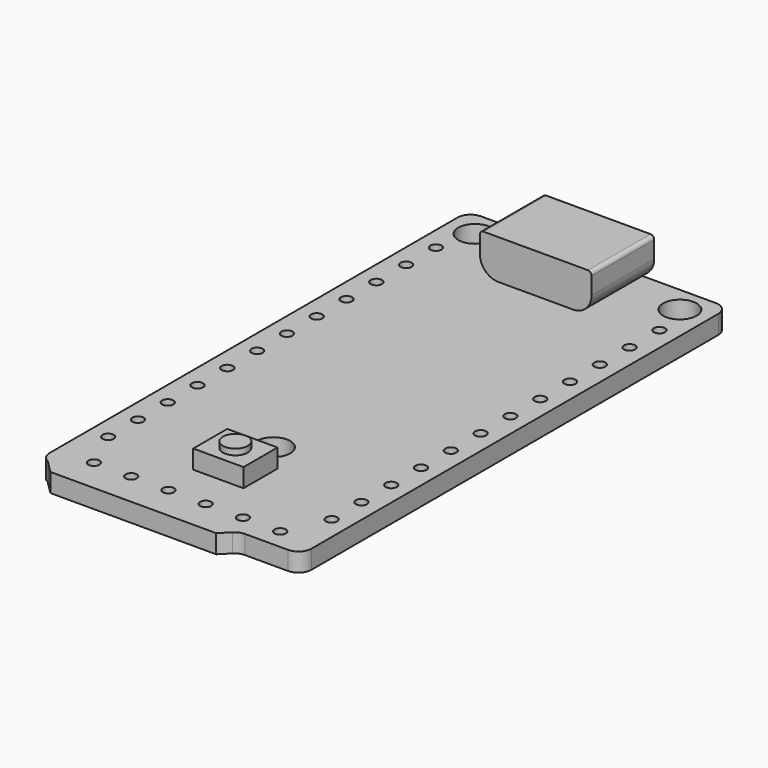
from build123d import *

# Parameters (mm, degrees)
F0_W        = 17.78
F0_H        = 37.338
F1_DEPTH    = 1.27
F2_R        = 1.143
F3_DEPTH    = 1.27
F5_DEPTH    = 25.4
F6_T1_DEPTH = 1.27
F6_T3_DEPTH = 5.715
F6_T5_DEPTH = 5.715
F6_T7_DEPTH = 5.715
F6_T9_DEPTH = 5.2860926284
F8_DEPTH    = 5.334
F9_R        = 0.381
F10_DEPTH   = 1.27
F11_R       = 0.381
F12_DEPTH   = 1.27
F14_DEPTH   = 4.953
F15_R       = 0.254
F16_W       = 3.429
F16_H       = 2.8956
F17_DEPTH   = 1.27
F18_R       = 0.8509
F19_DEPTH   = 0.4064


# Not quite as in the source:
# - a fillet or chamfer that OpenCascade refuses, or shapes differently, is made with other operations: its cross-section is extruded or revolved along the edge and cut away or added


with BuildPart() as f1:
    # F0 (on Top) → F1 (new body)
    with BuildSketch(Plane.XY):
        Rectangle(F0_W, F0_H)
    extrude(amount=F1_DEPTH)

    # F2 (on face) → F3 (cut, through all)
    with BuildSketch(Plane.XY.offset(1.27)):
        with Locations((6.985, 16.891)):
            Circle(F2_R)
        with Locations((-6.985, 16.891)):
            Circle(F2_R)
        with Locations((0, -9.017)):
            Circle(F2_R)
    extrude(amount=-F3_DEPTH, mode=Mode.SUBTRACT)

    # F4 (on face) → F5 (cut)
    with BuildSketch(Plane.XY.offset(1.27)):
        Polygon((-8.89, -17.78), (-8.89, -18.669), (-7.493, -18.669), (-8.382, -17.78), align=None)
        Polygon((8.89, -18.669), (8.89, -17.78), (4.699, -17.78), (3.81, -18.669), align=None)
    extrude(amount=-F5_DEPTH, mode=Mode.SUBTRACT)

    # F6: fillet of radius 0.889 on 5 edges, made by hand

    # F6_s2 → F6_t1 (join)
    with BuildSketch(Plane.XY):
        with BuildLine():
            ThreePointArc((5.0672358569, -17.78), (4.7270302856, -17.8476710956), (4.4386179285, -18.0403820715))
            Line((4.4386179285, -18.0403820715), (4.699, -17.78))
            Line((4.699, -17.78), (5.0672358569, -17.78))
        make_face()
    extrude(amount=F6_T1_DEPTH)

    # F6_s4 → F6_t3 (cut)
    with BuildSketch(Plane.XY.offset(-2.2225)):
        with BuildLine():
            ThreePointArc((8.001, 18.669), (8.6296179285, 18.4086179285), (8.89, 17.78))
            Line((8.89, 17.78), (8.89, 18.669))
            Line((8.89, 18.669), (8.001, 18.669))
        make_face()
    extrude(amount=F6_T3_DEPTH, mode=Mode.SUBTRACT)

    # F6_s6 → F6_t5 (cut)
    with BuildSketch(Plane.XY.offset(-2.2225)):
        with BuildLine():
            ThreePointArc((-8.001, 18.669), (-8.6296179285, 18.4086179285), (-8.89, 17.78))
            Line((-8.89, 17.78), (-8.89, 18.669))
            Line((-8.89, 18.669), (-8.001, 18.669))
        make_face()
    extrude(amount=F6_T5_DEPTH, mode=Mode.SUBTRACT)

    # F6_s8 → F6_t7 (cut)
    with BuildSketch(Plane.XY.offset(-2.2225)):
        with BuildLine():
            ThreePointArc((8.001, -17.78), (8.6296179285, -17.5196179285), (8.89, -16.891))
            Line((8.89, -16.891), (8.89, -17.78))
            Line((8.89, -17.78), (8.001, -17.78))
        make_face()
    extrude(amount=F6_T7_DEPTH, mode=Mode.SUBTRACT)

    # F6_s10 → F6_t9 (cut)
    with BuildSketch(Plane.XY.offset(-2.0080463142)):
        with BuildLine():
            ThreePointArc((-8.382, -17.78), (-8.7523421325, -17.4519719624), (-8.89, -16.9767814743))
            Line((-8.89, -16.9767814743), (-8.89, -17.78))
            Line((-8.89, -17.78), (-8.382, -17.78))
        make_face()
    extrude(amount=F6_T9_DEPTH, mode=Mode.SUBTRACT)

    # F7 (on face) → F8 (join)
    with BuildSketch(Plane(origin=(0, 18.669, 0), x_dir=(-1, 0, 0), z_dir=(0, 1, 0))):
        with BuildLine():
            Line((3.81, 3.9624), (0, 3.9624))
            Line((0, 3.9624), (-3.81, 3.9624))
            Line((-3.81, 3.9624), (-3.81, 2.54))
            ThreePointArc((-3.81, 2.54), (-3.4380256121, 1.6419743879), (-2.54, 1.27))
            Line((-2.54, 1.27), (0, 1.27))
            Line((0, 1.27), (2.54, 1.27))
            ThreePointArc((2.54, 1.27), (3.4380256121, 1.6419743879), (3.81, 2.54))
            Line((3.81, 2.54), (3.81, 3.9624))
        make_face()
    extrude(amount=-F8_DEPTH)

    # F9 (on face) → F10 (cut, through all)
    with BuildSketch(Plane.XY.offset(1.27)):
        with Locations((7.62, 14.351)):
            Circle(F9_R)
        with Locations((7.62, 11.811)):
            Circle(F9_R)
        with Locations((7.62, 9.271)):
            Circle(F9_R)
        with Locations((7.62, 6.731)):
            Circle(F9_R)
        with Locations((7.62, 4.191)):
            Circle(F9_R)
        with Locations((7.62, 1.651)):
            Circle(F9_R)
        with Locations((7.62, -0.889)):
            Circle(F9_R)
        with Locations((7.62, -3.429)):
            Circle(F9_R)
        with Locations((7.62, -5.969)):
            Circle(F9_R)
        with Locations((7.62, -8.509)):
            Circle(F9_R)
        with Locations((7.62, -11.049)):
            Circle(F9_R)
        with Locations((7.62, -13.589)):
            Circle(F9_R)
        with Locations((-7.62, -13.589)):
            Circle(F9_R)
        with Locations((-7.62, -11.049)):
            Circle(F9_R)
        with Locations((-7.62, -8.509)):
            Circle(F9_R)
        with Locations((-7.62, -5.969)):
            Circle(F9_R)
        with Locations((-7.62, -3.429)):
            Circle(F9_R)
        with Locations((-7.62, -0.889)):
            Circle(F9_R)
        with Locations((-7.62, 1.651)):
            Circle(F9_R)
        with Locations((-7.62, 4.191)):
            Circle(F9_R)
        with Locations((-7.62, 6.731)):
            Circle(F9_R)
        with Locations((-7.62, 9.271)):
            Circle(F9_R)
        with Locations((-7.62, 11.811)):
            Circle(F9_R)
        with Locations((-7.62, 14.351)):
            Circle(F9_R)
    extrude(amount=-F10_DEPTH, mode=Mode.SUBTRACT)

    # F11 (on face) → F12 (cut, through all)
    with BuildSketch(Plane.XY.offset(1.27)):
        with Locations((-6.35, -16.383)):
            Circle(F11_R)
        with Locations((-3.81, -16.383)):
            Circle(F11_R)
        with Locations((-1.27, -16.383)):
            Circle(F11_R)
        with Locations((1.27, -16.383)):
            Circle(F11_R)
        with Locations((3.81, -16.383)):
            Circle(F11_R)
        with Locations((6.35, -16.383)):
            Circle(F11_R)
    extrude(amount=-F12_DEPTH, mode=Mode.SUBTRACT)

    # F13 (on face) → F14 (cut, through all)
    with BuildSketch(Plane(origin=(0, 18.669, 0), x_dir=(-1, 0, 0), z_dir=(0, 1, 0))):
        with BuildLine():
            Line((-2.54, 1.6509998994), (2.54, 1.6509998994))
            ThreePointArc((2.54, 1.6509998994), (3.1686179996, 1.9113820004), (3.4290001006, 2.54))
            Line((3.4290001006, 2.54), (3.4290001006, 3.5814001006))
            Line((3.4290001006, 3.5814001006), (-3.4290001006, 3.5814001006))
            Line((-3.4290001006, 3.5814001006), (-3.4290001006, 2.54))
            ThreePointArc((-3.4290001006, 2.54), (-3.1686179996, 1.9113820004), (-2.54, 1.6509998994))
        make_face()
    extrude(amount=-F14_DEPTH, mode=Mode.SUBTRACT)

    # F15
    f15_edges = [f1.edges().sort_by_distance(p)[0] for p in [
        (3.81, 16.002, 3.9624),
        (-3.81, 16.002, 3.9624),
    ]]
    fillet(f15_edges, radius=F15_R)

    # F16 (on face) → F17 (join)
    with BuildSketch(Plane.XY.offset(1.27)):
        with Locations((0, -12.2682)):
            Rectangle(F16_W, F16_H)
    extrude(amount=F17_DEPTH)

    # F18 (on face) → F19 (join)
    with BuildSketch(Plane.XY.offset(2.54)):
        with Locations((0, -12.2682)):
            Circle(F18_R)
    extrude(amount=F19_DEPTH)


solid = f1.part
